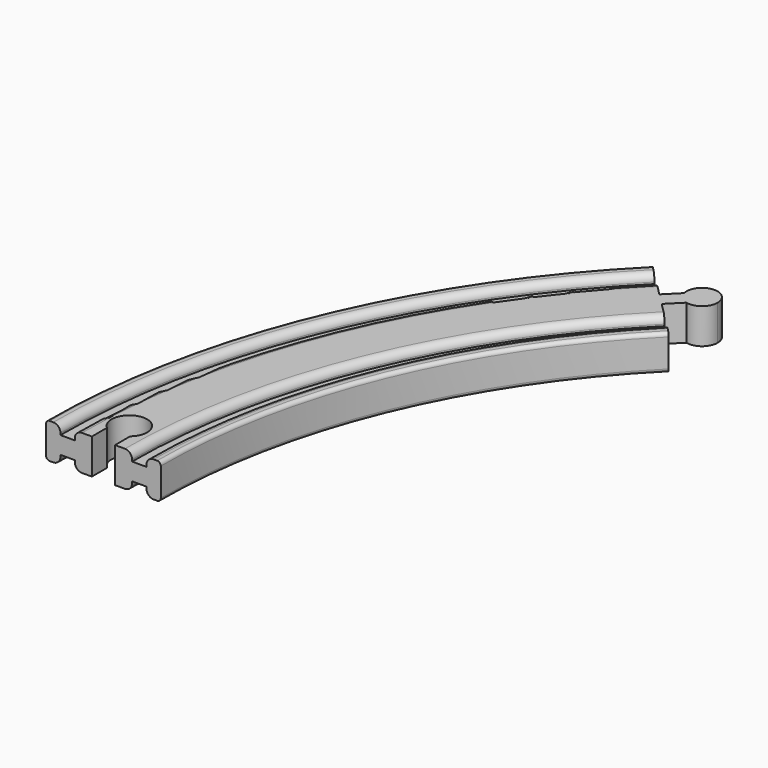
from build123d import *

# Parameters (mm, degrees)
F1_DEPTH  = 12.5
F3_DEPTH  = 12.501
F5_DEPTH  = 3.175
F7_R      = 1.27
F8_R      = 2.54
F10_DEPTH = 12.5


# Not quite as in the source:
# - a pattern or mirror of a feature is missing from the dataset's text; its kind, count and spacing are read off the source's solid


with BuildPart() as f1:
    # F0 (on Top) → F1 (new body)
    with BuildSketch(Plane.XY):
        with BuildLine():
            Line((-148.0681599805, 148.0681599805), (-176.7766952966, 176.7766952966))
            ThreePointArc((-176.7766952966, 176.7766952966), (-230.9698831278, 95.6708580913), (-250, 0))
            Line((-250, 0), (-209.4, 0))
            ThreePointArc((-209.4, 0), (-193.4603741079, 80.1339107372), (-148.0681599805, 148.0681599805))
        make_face()
    extrude(amount=F1_DEPTH)

    # F2 (on face) → F3 (cut, through all)
    with BuildSketch(Plane.XY.offset(12.5)):
        with BuildLine():
            Line((-225.6, 0), (-225.6, 6.6966957028))
            ThreePointArc((-225.6, 6.6966957028), (-229.7, 17.78), (-233.8, 6.6966957028))
            Line((-233.8, 6.6966957028), (-233.8, 0))
            Line((-233.8, 0), (-229.7, 0))
            Line((-229.7, 0), (-225.6, 0))
        make_face()
    extrude(amount=-F3_DEPTH, mode=Mode.SUBTRACT)

    # F4 (on face) → F5 (cut)
    with BuildSketch(Plane.XY.offset(12.5)):
        with BuildLine():
            Line((-169.5924903998, 169.5924903998), (-173.1845928482, 173.1845928482))
            ThreePointArc((-173.1845928482, 173.1845928482), (-226.2765751027, 93.7268262549), (-244.92, 0))
            Line((-244.92, 0), (-239.84, 0))
            ThreePointArc((-239.84, 0), (-221.5832670775, 91.7827944184), (-169.5924903998, 169.5924903998))
        make_face()
        with BuildLine():
            ThreePointArc((-214.48, 0), (-198.153682133, 82.0779425737), (-151.6602624289, 151.6602624289))
            Line((-151.6602624289, 151.6602624289), (-155.2523648773, 155.2523648773))
            ThreePointArc((-155.2523648773, 155.2523648773), (-202.8469901582, 84.0219744101), (-219.56, 0))
            Line((-219.56, 0), (-214.48, 0))
        make_face()
    f5 = extrude(amount=-F5_DEPTH, mode=Mode.SUBTRACT)

    # F5_copies: F5 across plane
    add(f5.mirror(Plane(origin=(0, 0, 6.25), x_dir=(-1, 0, 0), z_dir=(0, 0, -1))), mode=Mode.SUBTRACT)

    # F7
    f7_edges = [f1.edges().sort_by_distance(p)[0] for p in [
        (-230.969883, 95.670858, 12.5),
        (-193.460374, 80.133911, 12.5),
        (-193.460374, 80.133911, 0),
        (-230.969883, 95.670858, 0),
    ]]
    fillet(f7_edges, radius=F7_R)

    # F8
    f8_edges = [f1.edges().sort_by_distance(p)[0] for p in [
        (-226.276575, 93.726826, 12.5),
        (-198.153682, 82.077943, 12.5),
        (-221.583267, 91.782794, 12.5),
        (-202.84699, 84.021974, 12.5),
        (-198.153682, 82.077943, 0),
        (-202.84699, 84.021974, 0),
        (-221.583267, 91.782794, 0),
        (-226.276575, 93.726826, 0),
    ]]
    fillet(f8_edges, radius=F8_R)

    # F9 (on face) → F10 (join, through all)
    with BuildSketch(Plane.XY.offset(12.5)):
        with BuildLine():
            ThreePointArc((-155.5378591224, 165.2411321629), (-150.8497482914, 166.2707245903), (-148.7553443158, 170.5895109613))
            ThreePointArc((-148.7553443158, 170.5895109613), (-154.9010674024, 176.0514741336), (-159.6037231142, 169.3069961547))
            ThreePointArc((-159.6037231142, 169.3069961547), (-158.1444316124, 166.7004236647), (-155.5378591224, 165.2411321629))
        make_face()
        with BuildLine():
            ThreePointArc((-155.5378591224, 165.2411321629), (-158.1444316124, 166.7004236647), (-159.6037231142, 169.3069961547))
            Line((-159.6037231142, 169.3069961547), (-164.4553596345, 164.4553596345))
            Line((-164.4553596345, 164.4553596345), (-162.4224276386, 162.4224276386))
            Line((-162.4224276386, 162.4224276385), (-160.3894956426, 160.3894956426))
            Line((-160.3894956426, 160.3894956426), (-155.5378591224, 165.2411321629))
        make_face()
    extrude(amount=-F10_DEPTH)


solid = f1.part
